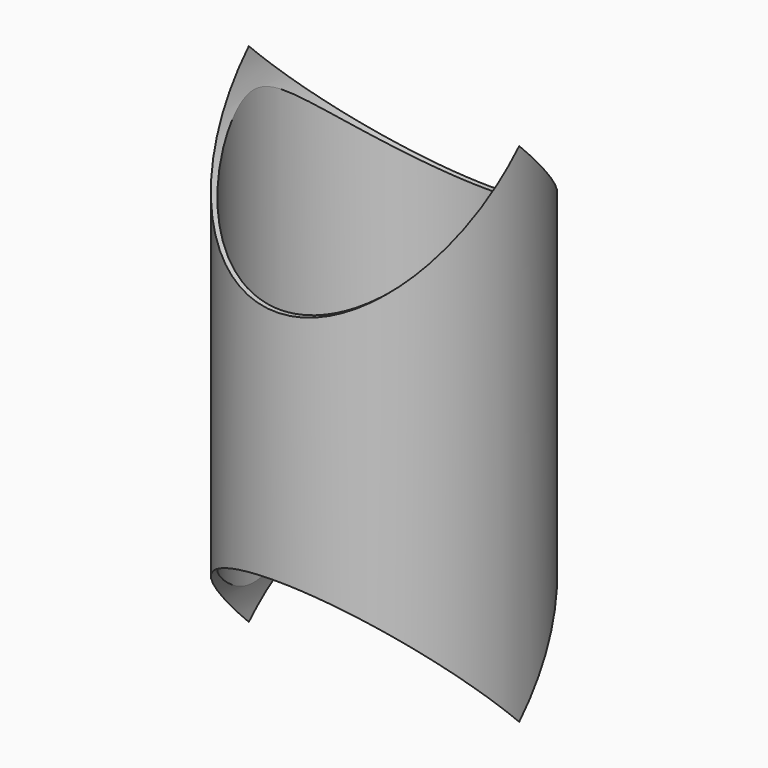
from build123d import *

# Parameters (mm, degrees)
F0_R          = 40
F0_R_2        = 38.5
F1_DEPTH      = 75
F2_R          = 40
F3_DEPTH      = 40.001
F3_DEPTH_BACK = 40.001


with BuildPart() as f1:
    # F0 (on Top) → F1 (new body, symmetric)
    with BuildSketch(Plane.XY):
        Circle(F0_R)
        Circle(F0_R_2, mode=Mode.SUBTRACT)
    extrude(amount=F1_DEPTH, both=True)

    # F2 (on Front) → F3 (cut, two sides)
    with BuildSketch(Plane.XZ) as f3_sk:
        with Locations((0, 75)):
            Circle(F2_R)
        with Locations((0, -75)):
            Circle(F2_R)
    extrude(amount=-F3_DEPTH, mode=Mode.SUBTRACT)
    extrude(f3_sk.sketch, amount=F3_DEPTH_BACK, mode=Mode.SUBTRACT)


solid = f1.part
